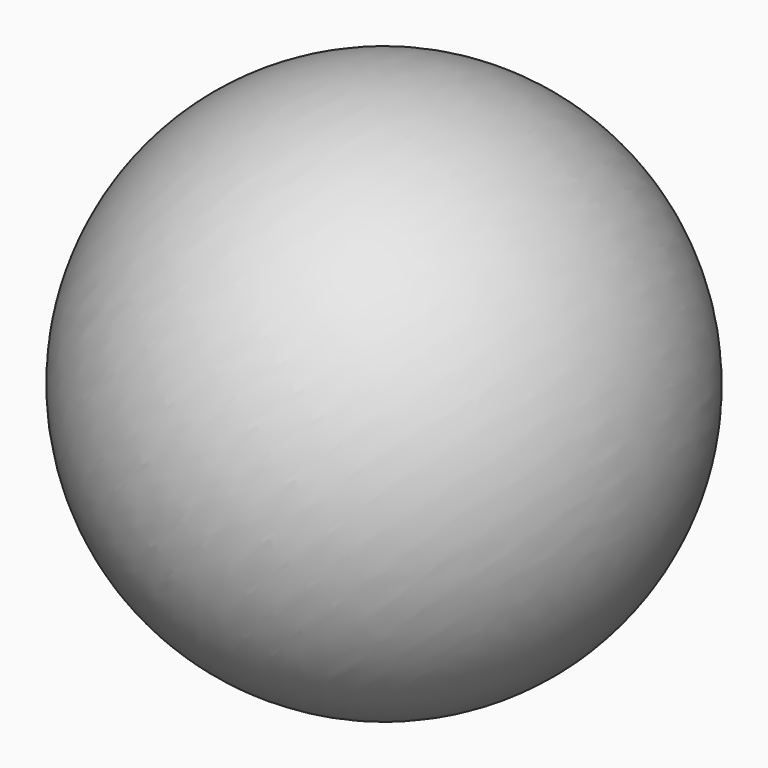
from build123d import *


with BuildPart() as f2:
    # F0 (on Front) → F2 (revolve)
    with BuildSketch(Plane.XZ):
        with BuildLine():
            Line((0, 0), (469.7830333099, -110.4837617667))
            ThreePointArc((469.7830333099, -110.4837617667), (110.4837617667, 469.7830333099), (-469.7830333099, 110.4837617667))
            Line((-469.7830333099, 110.4837617667), (0, 0))
        make_face()
    revolve(axis=Axis((-234.891516655, 0, 55.2418808834), (-0.9734418427, 0, 0.2289344421)))

    # F1 (on face) → F3 (revolve)
    with BuildSketch(Plane.XZ):
        with BuildLine():
            ThreePointArc((-361.8547041576, 356.5461724363), (296.0144982661, 412.843089825), (453.8106766266, -228.2977656038))
            Line((453.8106766266, -228.2977656038), (3.028395998, -1.5234900264))
            Line((3.028395998, -1.5234900264), (381.4318148132, -372.8610071438))
            ThreePointArc((381.4318148132, -372.8610071438), (373.5995359965, 380.7084799465), (-379.9837151417, 374.3366616124))
            Line((-379.9837151417, 374.3366616124), (-361.8547041576, 356.5461724363))
        make_face()
    revolve(axis=Axis((0.7240498358, 0, 0.7378272343), (-0.7137391825, 0, 0.7004115785)))


solid = f2.part
